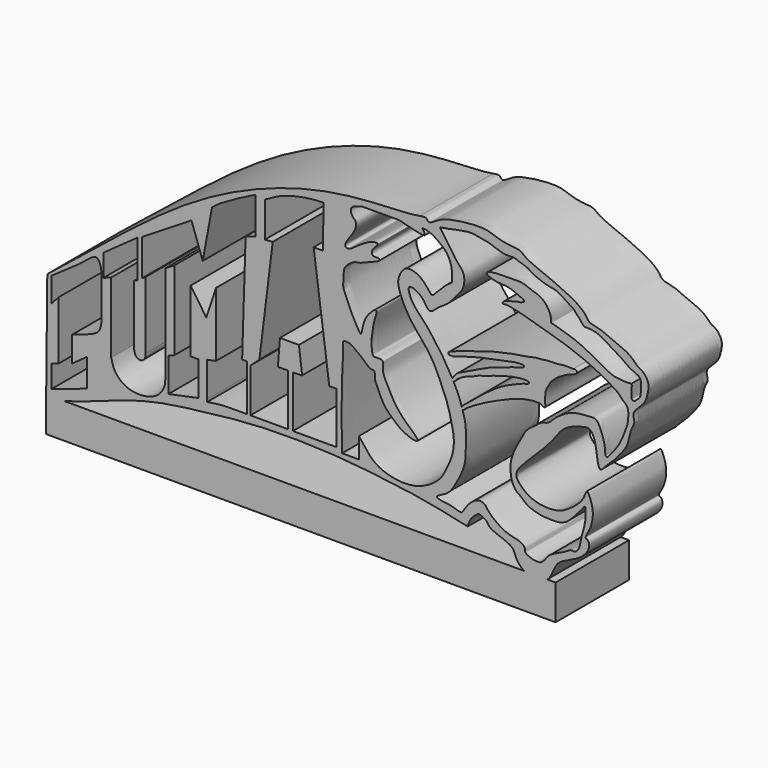
from build123d import *

# Parameters (mm, degrees)
F1_DEPTH = 20
F2_W     = 111.0479156588
F2_H     = 7.6344155701
F3_DEPTH = 20


with BuildPart() as f1:
    # F0 (on Front) → F1 (new body)
    with BuildSketch(Plane.XZ):
        with BuildLine():
            add(Edge.make_bspline(
                [(-68.5763731599, -24.029718712), (-62.8424740639, -19.4761018218), (-51.2870427359, -9.9741760052), (-32.577207567, 3.8970302083), (-8.5290191206, 12.8961252081), (9.7086163121, 13.0013621624), (12.0042391692, 13.4216141178), (12.6355951652, 13.5370446369)],
                knots=[0, 0, 0, 0, 0.2305075204, 0.4671476986, 0.7203497781, 0.9230047089, 1, 1, 1, 1], degree=3))
            Line((-68.5763731599, -24.029718712), (-68.8400990123, -49.0021140309))
            Line((-68.8400990123, -49.0021140309), (-67.2818273306, -47.8710122406))
            add(Edge.make_bspline(
                [(-67.2818273306, -47.8710122406), (-61.0936873368, -46.3664774949), (-49.1456948203, -41.1773982467), (-35.9901500826, -39.5859325488), (-23.4933828008, -38.0194479617), (-7.9544184747, -38.0854578186), (4.0351011583, -39.3360079001), (13.9875895572, -40.6665019925), (20.1001078469, -42.0224792595), (23.0631544298, -42.6801430644)],
                knots=[0, 0, 0, 0, 0.1748702622, 0.3187366349, 0.459197766, 0.6158479055, 0.754475325, 0.8794420979, 1, 1, 1, 1], degree=3))
            ThreePointArc((23.0631544298, -42.6801430644), (23.9464490144, -40.7759790038), (25.5563499174, -39.429030907))
            add(Edge.make_bspline(
                [(25.5563499174, -39.429030907), (26.1716625414, -39.6596022431), (27.3518612756, -40.1044976448), (27.7137964068, -41.7947097929), (33.1747303772, -42.9476295263), (33.3915021172, -45.4281539159), (35.7692568103, -48.0598457762), (41.3055342618, -47.9927628403), (41.9812373993, -42.883346931), (46.4047970825, -41.7440891079), (49.7857335986, -38.9620867614), (49.4956044988, -36.6956066003), (48.363130973, -36.5804430799), (49.9309341811, -34.6064106874), (50.5213747284, -31.4169708175), (50.108031679, -29.3425503211), (49.0232752449, -26.6090951701), (48.4739110603, -29.5594445155), (45.1258995017, -32.2008787119), (42.6546621411, -33.4876654823), (38.9384909011, -33.4863281815), (36.339694077, -32.5510247197), (34.2587013719, -30.8460209421), (33.14465329, -28.8158671071), (36.3034997793, -25.5921561608), (39.625862845, -22.3717114064), (41.6447003496, -20.0915280792), (43.0394886465, -17.9829548722), (44.9649642471, -16.270024253), (48.1341514666, -15.3318192091), (49.8205409339, -15.0591641924), (51.2193543877, -17.5815222843), (51.4579236491, -23.513175539), (53.1785046157, -21.1480303175), (54.7164859754, -19.9741312742), (56.5790834553, -17.6703813705), (58.1932679013, -15.5653781875), (58.4560193303, -12.5331844032), (59.7591870259, -10.8853380525), (58.5829563084, -9.0027633437), (61.709761443, -6.8157320682), (62.2784459421, -4.5471949838), (62.7867288075, -2.1367958021), (61.0445580767, -0.2100928655), (60.2541340875, -0.0851524026), (59.4746538103, 0.7961116283), (57.9762840665, 2.1258575397), (54.7069320423, 3.3546083874), (52.2854621802, 4.6056235075), (49.4149561727, 4.9542350847), (48.9835662994, 6.2526229564), (46.680608127, 8.2529520546), (43.1362195894, 9.7788813803), (41.6027546429, 10.5205784164), (39.6470245398, 11.3299557773), (37.4213779274, 12.1396946885), (35.4958827322, 13.1736840083), (34.3536675322, 14.2578538304), (31.7790832126, 14.2057000076), (28.8726627219, 15.0299179873), (27.1131732469, 15.7523169184), (23.3109314875, 15.6544083262), (19.399034179, 15.0975749866), (16.7432067765, 14.2594341947), (14.9146380272, 12.8093572388), (14.2668846406, 13.1623013209), (14.0411098054, 13.7738687719), (13.1720313766, 13.627432199), (12.6355951652, 13.5370446369)],
                knots=[0, 0, 0, 0, 0.0128906595, 0.0246453603, 0.0460755988, 0.0603354354, 0.0777175692, 0.0981562797, 0.1177821882, 0.1378619387, 0.1576052625, 0.170275515, 0.1777469708, 0.19122827, 0.2088810173, 0.2238704146, 0.236935849, 0.2498612246, 0.2700920494, 0.286410647, 0.3045313212, 0.3206836367, 0.3363322107, 0.3493730315, 0.3688889221, 0.3903022143, 0.407043062, 0.4220983379, 0.4376305213, 0.4551207774, 0.4665194786, 0.4826922908, 0.5034058812, 0.5151812999, 0.5294625771, 0.5458845909, 0.5616833513, 0.5782965055, 0.5915054006, 0.6038100797, 0.6213156282, 0.6362732181, 0.6510407179, 0.665696027, 0.6740429806, 0.6839305184, 0.6976067432, 0.7155841904, 0.7321442087, 0.7476178336, 0.7579985815, 0.7747019213, 0.7938175182, 0.8064582323, 0.8202405581, 0.8353452595, 0.8495036912, 0.8611660563, 0.8763967251, 0.893141174, 0.9064170318, 0.92499084, 0.944463415, 0.9608928393, 0.9748715551, 0.981946496, 0.9888043556, 1, 1, 1, 1], degree=3))
        make_face()
        with BuildLine():
            Line((-67.6202252507, -29.3487161398), (-67.6202252507, -24.029718712))
            add(Edge.make_bspline(
                [(-63.15773819, -33.9078567922), (-61.5074046053, -33.3753877232), (-58.8261670773, -32.5103088081), (-57.1355470776, -31.3741286232), (-56.6463044332, -29.3712492055), (-56.7989735672, -25.0925295019), (-56.5854431257, -19.2767948952), (-57.3062910621, -17.7206121949), (-58.1642828184, -17.0182992197), (-60.3673849688, -18.9638502975), (-64.6799909941, -22.1019544197), (-67.6202252507, -24.029718712)],
                knots=[0, 0, 0, 0, 0.1344522729, 0.21810492, 0.301110973, 0.4329190842, 0.5837822348, 0.6615185097, 0.714935113, 0.8099422179, 1, 1, 1, 1], degree=3))
            Line((-63.15773819, -33.9078567922), (-63.15773819, -39.4494543357))
            Line((-63.15773819, -39.4494543357), (-59.9204339087, -37.0995940954))
            Line((-59.9204339087, -37.0995940954), (-59.9204339087, -43.2110093534))
            Line((-59.9204339087, -43.2110093534), (-67.681632936, -45.812278986))
            Line((-67.681632936, -45.812278986), (-67.681632936, -40.9478149984))
            Line((-67.681632936, -40.9478149984), (-66.1323964596, -40.4285676777))
            Line((-66.1323964596, -40.4285676777), (-66.1323964596, -27.7001184301))
            Line((-66.1323964596, -27.7001184301), (-67.6202252507, -29.3487161398))
        make_face(mode=Mode.SUBTRACT)
        with BuildLine():
            Line((-56.3480295241, -20.7848474383), (-56.3480295241, -15.9424301237))
            Line((-56.3480295241, -15.9424301237), (-48.9367544651, -10.6603609944))
            Line((-48.9367544651, -10.6603609944), (-48.9367544651, -18.8947413117))
            Line((-48.9367544651, -18.8947413117), (-49.6612451971, -19.1793628672))
            Line((-49.6612451971, -19.1793628672), (-49.6612451971, -32.3095694184))
            add(Edge.make_bspline(
                [(-49.6612451971, -32.3095694184), (-49.550913704, -32.5792308171), (-49.4735777947, -33.3253336595), (-48.9232087266, -33.8958631419), (-47.8595334721, -34.0964704749), (-47.1028458665, -33.0518824561), (-47.1613099679, -32.5387496049), (-47.1861027181, -32.3095694184)],
                knots=[0, 0, 0, 0, 0.2109435836, 0.3940078694, 0.5974043108, 0.8207649572, 1, 1, 1, 1], degree=3))
            Line((-47.1861027181, -32.3095694184), (-47.1861027181, -17.6569670439))
            Line((-47.1861027181, -17.6569670439), (-47.9423962533, -18.1223899126))
            Line((-47.9423962533, -18.1223899126), (-47.9423962533, -10.2101974189))
            Line((-47.9423962533, -10.2101974189), (-37.1425785124, -3.4970382694))
            Line((-37.1425785124, -3.4970382694), (-34.6929617226, -10.4895886034))
            Line((-34.6929617226, -10.4895886034), (-32.6580479741, 0.4966819542))
            add(Edge.make_bspline(
                [(-32.6580479741, 0.4966819542), (-31.6459829579, 1.3301714982), (-29.8156036109, 2.5123849062), (-26.2045528268, 4.4330040138), (-24.1211841262, 5.55334523), (-23.2389662415, 5.9331734665)],
                knots=[0, 0, 0, 0, 0.3299609283, 0.6827711276, 1, 1, 1, 1], degree=3))
            Line((-23.2389662415, 5.9331734665), (-23.2389662415, -2.0397095941))
            Line((-23.2389662415, -2.0397095941), (-25.3467336297, -2.7791610919))
            Line((-25.3467336297, -2.7791610919), (-26.1013221078, -26.6294348985))
            Line((-26.1013221078, -26.6294348985), (-25.0671431422, -26.6294348985))
            Line((-25.0671431422, -26.6294348985), (-25.0671431422, -36.741334945))
            add(Edge.make_bspline(
                [(-25.0671431422, -36.741334945), (-26.3252303884, -36.7258496034), (-28.7008392181, -36.6966090922), (-31.6308565733, -36.8875220527), (-33.0835662989, -37.1412270736), (-33.7508358061, -37.2577607632)],
                knots=[0, 0, 0, 0, 0.378372384, 0.7144693495, 1, 1, 1, 1], degree=3))
            Line((-33.7508358061, -37.2577607632), (-33.7640754879, -36.741334945))
            Line((-33.7640754879, -36.741334945), (-33.7640754879, -29.138345798))
            Line((-33.7640754879, -29.138345798), (-31.794089824, -28.7411157042))
            Line((-31.794089824, -28.7411157042), (-31.794089824, -14.7206289694))
            Line((-31.794089824, -14.7206289694), (-33.918403089, -21.0935790092))
            Line((-33.918403089, -21.0935790092), (-37.3236909509, -16.0667231292))
            Line((-37.3236909509, -16.0667231292), (-37.3236909509, -29.6698175371))
            Line((-37.3236909509, -29.6698175371), (-35.660982132, -29.6698175371))
            Line((-35.660982132, -29.6698175371), (-35.660982132, -37.109284196))
            Line((-35.660982132, -37.109284196), (-42.1798937023, -38.4673907732))
            Line((-42.1798937023, -38.4673907732), (-42.1798937023, -31.0817323625))
            Line((-42.1798937023, -31.0817323625), (-40.8984795213, -30.6096319109))
            Line((-40.8984795213, -30.6096319109), (-40.8984795213, -13.3854517873))
            Line((-40.8984795213, -13.3854517873), (-42.8405329585, -14.5506840199))
            Line((-42.8405329585, -14.5506840199), (-42.8405329585, -35.5389267206))
            add(Edge.make_bspline(
                [(-54.6512380242, -35.5389267206), (-54.4245839545, -36.4442620263), (-53.931170017, -38.415129165), (-50.5420565368, -40.9685900651), (-45.2064643534, -40.5118258501), (-42.9223532416, -37.8091151365), (-42.8659685902, -36.2446646398), (-42.8405329585, -35.5389267206)],
                knots=[0, 0, 0, 0, 0.1836112314, 0.3997119522, 0.644773585, 0.8397541172, 1, 1, 1, 1], degree=3))
            Line((-54.6512380242, -35.5389267206), (-54.6512380242, -20.1670583338))
            Line((-54.6512380242, -20.1670583338), (-56.3480295241, -20.7848474383))
        make_face(mode=Mode.SUBTRACT)
        with BuildLine():
            Line((-21.1528521031, -2.0069417078), (-21.1528521031, 5.7083428837))
            add(Edge.make_bspline(
                [(-21.1528521031, 5.7083428837), (-20.1003651535, 6.3187885742), (-17.9155580527, 7.5859834595), (-13.7988873339, 8.7460943954), (-10.4805822381, 9.2007744218), (-9.0379980514, 9.2152428669), (-8.4088556468, 9.2215528712)],
                knots=[0, 0, 0, 0, 0.2663248992, 0.5528510649, 0.8049886039, 1, 1, 1, 1], degree=3))
            Line((-8.4088556468, 9.2215528712), (-8.4274644032, 0))
            Line((-8.4274644032, 0), (-10.5071477592, 0))
            Line((-10.5071477592, 0), (-7.1003274061, -25.5388338119))
            Line((-7.1003274061, -25.5388338119), (-5.4923477583, -25.5388338119))
            Line((-5.4923477583, -25.5388338119), (-5.4923477583, -36.741334945))
            Line((-5.4923477583, -36.741334945), (-15.0402951986, -36.741334945))
            Line((-15.0402951986, -36.741334945), (-15.0402951986, -25.47673136))
            Line((-15.0402951986, -25.47673136), (-13.0293034017, -25.410797447))
            Line((-13.0293034017, -25.410797447), (-13.7177789584, -19.7872146964))
            Line((-13.7177789584, -19.7872146964), (-17.861418426, -19.7872146964))
            Line((-17.861418426, -19.7872146964), (-18.3040369302, -25.47673136))
            Line((-18.3040369302, -25.47673136), (-16.0689745098, -25.47673136))
            Line((-16.0689745098, -25.47673136), (-16.0689745098, -36.741334945))
            Line((-16.0689745098, -36.741334945), (-24.2825746536, -36.741334945))
            Line((-24.2825746536, -36.741334945), (-24.2825746536, -27.1698180586))
            Line((-24.2825746536, -27.1698180586), (-22.335955239, -25.410797447))
            Line((-22.335955239, -25.410797447), (-19.4306913763, -1.869168831))
            Line((-19.4306913763, -1.869168831), (-21.1528521031, -2.0069417078))
        make_face(mode=Mode.SUBTRACT)
        with BuildLine():
            add(Edge.make_bspline(
                [(13.1149329245, 11.4469267428), (13.2454424113, 11.265540442), (13.5017344209, 10.9093375275), (14.0798250427, 9.9265843409), (11.9921920887, 10.3150667891), (9.3961707003, 10.8682942314), (8.3365435753, 11.3562675048), (5.2628460876, 11.1676267303), (1.4134467959, 11.2473589646), (0.0227734326, 11.3111626559), (-0.8636605807, 10.8570442048), (-1.9383073615, 10.6542583041), (-2.4270764263, 10.1920794525), (-2.4098521462, 9.325496849), (-1.936654468, 8.4605651843), (-1.2957633129, 8.1106285788), (-1.1941500149, 6.5018633305), (-2.3064935859, 5.0299367339), (-3.2934459387, 3.6039608268), (-3.7530027477, 2.6985577325), (-3.363455326, 2.0513797894), (-2.2784933492, 2.3048448469), (-0.6581018721, 3.7386091033), (1.1914715646, 4.671528638), (2.0996055947, 5.2467896361), (4.0963186692, 5.4843413959), (2.4310462008, 3.9496448812), (2.057302188, 3.2403916948), (2.4101538771, 2.334543307), (3.6449311374, 2.5977628138), (3.9979083618, 2.2141175488), (3.3495048099, 1.6984931235), (1.7460088106, 1.2415812933), (-0.3552107945, 0.1699458693), (-1.698762065, 0.1970740724), (-3.4454235187, -1.1434876811), (-4.0011264115, -2.1229225594), (-4.0193230978, -4.5170312493), (-4.1669284386, -5.7428791166), (-2.8987263025, -8.3243099324), (-2.1297921371, -10.3240843808), (-0.6548038421, -12.8414710721), (-0.2276660592, -13.4580342627), (0.0556774798, -12.6325087625), (0.2337403686, -11.4435931249), (0.6618419334, -10.2191982524), (1.269346609, -9.1390326043), (2.1484826433, -8.231889505), (2.5779945286, -7.8418971873), (2.8517618261, -7.6601574257), (3.1762750434, -7.5546178135), (3.2616173012, -8.2027558151), (2.7811510965, -9.4209664527), (2.4302861584, -10.9923666744), (2.2550789719, -12.4495099501), (2.0075769976, -13.7766201014), (2.1885419282, -15.7747065486), (2.4751401995, -16.889099067), (3.4669993278, -16.6221565323), (4.2346679021, -16.7619717693), (4.7779826125, -17.0446088063), (4.3344533036, -19.0130874806), (5.721595114, -21.4741059315), (6.9664758787, -24.0776386974), (9.2151011375, -26.8092605363), (10.6988688311, -27.9292142464), (11.7172701448, -28.9657842684), (12.4404026364, -29.8329394905), (11.3742229698, -30.0095697484), (9.9356421891, -29.4498423173), (8.4618387431, -28.8139448721), (6.6323109237, -27.1865886424), (5.0062867854, -25.6943605934), (3.8998537977, -23.5413761077), (3.2636028786, -21.9867176539), (2.7069994861, -20.915651109), (2.9770063005, -19.252616312), (1.7969919761, -19.4229915113), (0.9098473053, -18.5047254773), (-0.6092325432, -17.2494448742), (-1.533446625, -16.6011797284), (-2.487423885, -15.8622744104), (-3.2908907548, -15.860254335), (-4.2504746017, -15.6163677239), (-4.019144832, -18.0375390004), (-4.3630860957, -22.2375592594), (-4.5214006905, -31.2084520815), (-4.3110004626, -37.5204570591)],
                knots=[0, 0, 0, 0, 0.0083871544, 0.0164688024, 0.0288112058, 0.0453967227, 0.0558365001, 0.0729670657, 0.0926563772, 0.1039508445, 0.1135550149, 0.1237527145, 0.13132907, 0.1401639553, 0.1497659263, 0.1577698247, 0.1693629384, 0.1828971777, 0.1960573939, 0.2055387359, 0.2127473388, 0.2221709698, 0.2369159506, 0.2510110489, 0.2619725466, 0.2725744132, 0.2847141685, 0.2940190896, 0.3022983772, 0.3127711078, 0.318330634, 0.3260539625, 0.3391321531, 0.3541499816, 0.3656172875, 0.3796016841, 0.3902381501, 0.4050102041, 0.4162654288, 0.4323176585, 0.4477357949, 0.4645012583, 0.4710358037, 0.4787105679, 0.4899162886, 0.5011140579, 0.5121907721, 0.5232303057, 0.5306436192, 0.5362746619, 0.5410445653, 0.5478224262, 0.5592434936, 0.5719266364, 0.5837295601, 0.5952873087, 0.6094166969, 0.6188578498, 0.627894564, 0.6366829551, 0.6432552251, 0.6562065851, 0.6727181209, 0.689834476, 0.7082012397, 0.72167869, 0.7337849309, 0.7424898352, 0.7507036997, 0.763097174, 0.7756890099, 0.7909391309, 0.8057673206, 0.8210006386, 0.833695512, 0.8446836397, 0.8559755358, 0.8648145789, 0.8758904082, 0.8897518873, 0.9004813451, 0.910936758, 0.9198801755, 0.927739317, 0.9408486915, 0.9609068341, 1, 1, 1, 1], degree=3))
            add(Edge.make_bspline(
                [(-0.6561594782, -33.0408181175), (-0.035652913, -33.8626542442), (1.2155842949, -35.5198674437), (3.5168527453, -37.8087591992), (7.9171780503, -39.0052123015), (11.7615988371, -38.7653015247), (14.5901260849, -37.533092362), (17.2156468794, -35.5901900018), (18.4976848628, -33.040918417), (19.8691271694, -30.1235870757), (20.2123975557, -26.7733900062), (19.5213175063, -23.6446639212), (18.6349047357, -20.2435125181), (17.6216857054, -17.9922458122), (15.6772356677, -13.3418208854), (13.2887033228, -10.2949847948), (10.7071343576, -7.3843904229), (8.8028686978, -4.1077386098), (7.7185245302, -1.0489519232), (8.1235728753, 0.8410546592), (9.4328177043, 2.799162206), (11.7395616106, 2.5336595786), (13.6792742589, 1.2327935868), (15.1922757938, -1.0484076658), (15.6880826756, -0.5522752558), (16.7707954606, 0.5779130569), (17.5241453321, 1.3605404433), (18.4301937149, 2.2307846442), (19.7242244397, 2.9620222635), (19.6149120897, 3.5342651834), (19.6917472385, 5.0038971788), (19.5024920618, 6.4153707199), (18.562032301, 8.497381305), (17.3070456925, 9.5000557411), (16.2776299305, 10.2762086716), (15.2740757169, 10.9309394715), (14.1412753371, 11.2924457196), (13.4495642164, 11.3966113586), (13.1149329245, 11.4469267428)],
                knots=[0, 0, 0, 0, 0.0322707381, 0.0650399499, 0.1038618123, 0.1398422198, 0.1719327954, 0.2045717184, 0.2354578959, 0.2683741304, 0.3017219568, 0.3349580476, 0.3688298157, 0.3981956437, 0.4389760175, 0.4757398142, 0.5117346155, 0.5479236801, 0.5803814755, 0.6055638571, 0.6320217353, 0.6579864657, 0.68734805, 0.7155466683, 0.7275571363, 0.7506067352, 0.7702509745, 0.7912750478, 0.8126057944, 0.8254268821, 0.8472173537, 0.8698461488, 0.8972195022, 0.9205493959, 0.9412780642, 0.9613483157, 0.9812982559, 1, 1, 1, 1], degree=3))
            Line((-0.6561594782, -33.0408181175), (-0.6561594782, -37.5204570591))
            Line((-0.6561594782, -37.5204570591), (-4.3110004626, -37.5204570591))
        make_face(mode=Mode.SUBTRACT)
        with BuildLine():
            add(Edge.make_bspline(
                [(17.0841336351, 12.7163172), (17.816161154, 11.6189452677), (19.1604477338, 9.6037474088), (20.6664432108, 7.3766720753), (22.3273993151, 5.8987675251), (22.3922207189, 3.6564091781), (21.8762247664, 2.0662007346), (19.8418630574, 0.0014335713), (18.8093748214, -1.4393306047), (16.5299443556, -2.6010367842), (14.7165509382, -4.7535042616), (13.5811906867, -2.2747865343), (12.2092411584, -1.2496068888), (11.0771416619, -0.6529574777), (9.8924641815, -0.7954449334), (10.6646527097, -3.1397247399), (11.9635149006, -4.8476877258), (14.0809259567, -6.8496355128), (16.4279645117, -10.0984268825), (17.6050110376, -11.769082258), (18.7496305182, -13.5767852663), (19.5360881146, -14.9832356329), (19.7466184679, -15.3735313595)],
                knots=[0, 0, 0, 0, 0.0093192229, 0.0171427526, 0.0240747115, 0.0308814227, 0.0370874622, 0.0450740315, 0.0514910318, 0.0592530711, 0.0661419814, 0.072887806, 0.079364404, 0.084724767, 0.0888693687, 0.0956151997, 0.1028282485, 0.1110450608, 0.1205682043, 0.1274133905, 0.135536896, 0.1385735761, 0.1385735761, 0.1385735761, 0.1385735761], degree=3))
            add(Edge.make_bspline(
                [(58.7086154351, -3.7098187022), (58.7575826978, -3.7638790664), (58.8801513344, -3.8991881436), (58.7910363742, -4.4402645372), (58.7984741188, -5.3751263327), (58.827958268, -6.2617494256), (58.7948619909, -6.6305001059), (59.023329139, -6.804572873), (59.419611634, -6.8195402864), (59.7205652029, -6.5973420149), (60.2618346637, -6.0927991422), (60.7810410992, -5.5238539958), (60.8377062719, -3.9874344052), (60.9149850635, -2.7600201737), (60.6335143592, -1.8824163864), (60.0588257828, -1.5117752223), (58.9051608413, -1.0406365304), (57.9045532683, -0.4783762414), (56.960296564, 0.2823810251), (56.372079104, 0.6558442358), (55.2364788399, 1.2875888185), (54.3585193901, 1.8877445624), (53.2848558449, 2.5497152391), (52.3615543424, 3.1321344463), (51.4897467898, 3.5136861858), (50.9092580092, 3.749535455), (50.1176164563, 3.8410651041), (49.1976692589, 3.9647302334), (48.6161478337, 3.8671370765), (48.3046605591, 4.1092904634), (47.8773003267, 4.4956294027), (47.4484080765, 5.2442345638), (46.740666053, 5.7640741683), (46.4357579422, 6.357542198), (45.8073218371, 6.810852867), (44.7552248108, 7.4451028528), (44.3673871829, 7.7093556556), (42.4701726692, 9.0448684169), (40.6611159434, 9.1058567867), (38.7132354371, 9.8441851555), (37.1997335101, 10.3881195268), (35.9960736002, 11.4177012251), (33.9643685252, 11.8495216408), (33.4325128393, 12.2505204309), (31.9566459365, 12.1783752773), (31.0754964675, 12.1965069011), (30.3087553781, 12.3822129666), (29.0440085637, 12.7601261379), (27.8975701844, 13.2911933304), (26.3540810585, 13.5165327709), (25.2937772269, 13.7127334798), (23.9007007887, 14.006713945), (22.0831354351, 13.7632054074), (20.3348467077, 13.4574687334), (19.0715778274, 13.0810325578), (17.7861806483, 12.9760156267), (17.2958679619, 12.7946453974), (17.0841336351, 12.7163172)],
                knots=[0, 0, 0, 0, 0.0086815097, 0.0217294282, 0.0400641548, 0.0575678905, 0.0681013381, 0.0771420047, 0.0882535158, 0.0993912764, 0.1150075426, 0.1309374985, 0.1534185133, 0.1743643813, 0.191119142, 0.2058959575, 0.2262785846, 0.2465590233, 0.266404454, 0.282005101, 0.302626303, 0.3220275248, 0.3425651169, 0.3620512832, 0.3797988096, 0.3942186767, 0.4106213396, 0.4285912517, 0.4422475538, 0.4531627477, 0.4669907378, 0.4841679055, 0.5013090904, 0.5158889746, 0.5323107728, 0.5522437279, 0.5655477651, 0.5924996252, 0.617961924, 0.6442183688, 0.6673603309, 0.6907647298, 0.7165811017, 0.7317131116, 0.7534632882, 0.7710177596, 0.7871074328, 0.8080429008, 0.8291476789, 0.8518529928, 0.8710599312, 0.8926616362, 0.9177481055, 0.942325045, 0.9636508351, 0.9843029605, 1, 1, 1, 1], degree=3))
            add(Edge.make_bspline(
                [(21.9570909853, -20.7023481974), (22.1617589553, -21.3451488475), (22.6255232655, -22.8545369616), (22.7628290276, -25.6850734761), (22.6044800653, -28.0524002222), (22.6630482648, -30.4810375624), (21.5756577584, -33.4289443176), (20.0774748785, -35.9052863937), (18.9399977193, -37.8942372624), (15.4264245939, -39.1611910228), (17.9375925547, -39.721482251), (19.5198153114, -39.7373460793), (21.7712222623, -40.7086491695), (22.1466773594, -39.8277220362), (23.1113128662, -38.4368667816), (24.0604874875, -37.5582384963), (25.2245033713, -36.7678866859), (26.773701419, -36.9661776917), (27.337202975, -38.0319782715), (28.5355602565, -39.2300801802), (29.7903036803, -40.1087975205), (31.3594197944, -41.0971273889), (32.9858494114, -41.4896303823), (34.785620179, -41.8553639259), (35.669664357, -42.7585421075), (35.4200260861, -43.6525324507), (36.6345797405, -44.133082294), (37.4080152648, -44.4595841819), (38.2734166908, -44.4398327569), (38.8863049383, -44.5017944242), (39.5539669693, -43.913984267), (39.9609931934, -43.6254855134), (40.4076708062, -42.6206470559), (42.0098513468, -41.6657050799), (43.3994366477, -41.0906560239), (44.785396748, -40.3213785416), (45.6164080501, -39.7677540186), (46.521235683, -40.0753950665), (47.2010057415, -39.2846746891), (47.5863294053, -38.4496625974), (47.7603901725, -36.7879551259), (48.3298418898, -35.2087307299), (48.5829920289, -33.9366407383), (48.8248997891, -32.6139479335), (48.7103626047, -31.3591021858), (48.8564791682, -30.6326217849), (48.5254651263, -30.4647876306), (48.1395884555, -31.1395609068), (47.5051630068, -31.7427461907), (46.6685071707, -32.838201186), (45.8140316113, -33.6537172631), (44.742550321, -34.7849723935), (43.7873997524, -35.1260370174), (43.1741337502, -35.4179251215), (41.8160349428, -35.4988036781), (40.5457155629, -35.4245411176), (39.134472636, -35.380796386), (37.881417918, -35.0319141641), (35.9338162559, -34.5023477853), (34.5922306293, -32.9525786188), (33.63937814, -32.5986030857), (32.7592339443, -31.115529487), (32.4586710582, -29.7401843279), (32.2696559612, -27.6786463417), (32.9518422537, -25.3892704061), (33.8239690305, -23.5770851636), (34.5318488814, -22.4781228728), (35.7189885129, -19.7652427926), (37.8928997811, -18.590705731), (39.0444794975, -17.3759520562), (40.7222385304, -17.2328282235), (41.8935065092, -15.7457985042), (43.6702551243, -14.4788553747), (45.3601794339, -13.520263261), (47.6249410087, -13.0104254186), (49.5398729125, -12.9804483669), (51.2136074746, -12.7141080475), (52.1251924565, -14.7361568064), (52.7086575632, -16.3746917208), (53.0762249851, -18.0843830926), (53.0422896471, -18.9931056505), (53.1158657774, -19.4635210054), (53.6816728465, -19.4550884439), (54.0061010095, -18.8387070718), (55.0555889082, -17.6514805797), (55.9463576285, -16.5062941165), (56.8954553882, -14.5585533584), (57.3412382773, -13.2828068298), (57.9441292253, -11.8173539235), (58.0609639819, -10.5692680316), (58.1402321195, -9.5256235493), (57.9583809654, -8.4775964297), (57.4685176773, -7.8970873717), (56.4808773462, -7.1451034441), (55.9651990755, -6.3409974695), (54.7425324129, -5.6311905423), (53.700542636, -4.9262028922), (52.0373160004, -3.9942087316), (50.5566739963, -3.3819793865), (48.4313147557, -2.2753733998), (46.7621464075, -1.8186019666), (44.7600525663, -0.9349911706), (43.0184715759, -0.3616440676), (40.0660248213, 0.4117238381), (38.9206011294, 0.8349585322), (37.19369387, 1.2552655679), (35.5683277256, 1.7441253504), (34.3198411783, 2.1256253149), (32.5317827325, 2.4056760321), (31.7233291036, 2.7301000951), (30.4397630983, 2.425161342), (30.9454199565, 3.2371337753), (31.813785914, 3.4477145651), (32.5207381284, 3.6538955757), (33.2678070342, 3.8194494394), (34.030521615, 4.064703185), (34.6223321118, 4.0591448265), (35.0683845205, 4.2955191024), (35.3944926818, 4.4514003975), (35.3626372612, 4.820600675), (34.6648119617, 5.0653313881), (33.8600526418, 5.4723733718), (33.0484340527, 5.8037602198), (31.9182266524, 6.1223758841), (30.7645751371, 6.285963445), (29.7105502774, 6.2660929675), (28.8708156015, 6.4612986785), (28.0946639595, 6.6666021541), (27.5831612412, 6.9748291234), (26.9632451016, 7.1638703367), (27.4622135024, 7.5956330707), (28.0324474284, 7.8062835435), (29.0695933516, 7.8943681245), (29.5886365979, 8.0016184079), (31.3452914813, 7.9513601066), (33.0337283392, 7.9969053119), (35.0875005651, 8.0779291486), (37.0152531251, 7.2188692107), (38.6184437488, 6.7633449226), (39.9123503189, 5.8758508046), (40.5178514487, 5.0144087489), (40.9631915911, 4.2483765607), (41.2853137372, 3.2676299862), (41.1874292427, 2.2056239193), (41.5571983026, 2.2824667118), (42.4420747207, 2.0632094857), (43.8452983351, 1.5362562125), (45.8290187598, 1.0533515843), (48.2710237653, -0.0028069515), (50.2076646979, -0.979686875), (52.8579240991, -2.5610829894), (54.0924406999, -3.1036408094), (54.8597335523, -3.4664090693), (55.8024361178, -3.5617820029), (57.151861267, -3.7312988694), (58.214317647, -3.7463954724), (58.5033871177, -3.6448721746), (58.7086154351, -3.7098187022)],
                knots=[0.154076916, 0.154076916, 0.154076916, 0.154076916, 0.1604338558, 0.1686540911, 0.1760206587, 0.1833923163, 0.1918310154, 0.1999162943, 0.2074824736, 0.2150247112, 0.2206649716, 0.2274229643, 0.234302321, 0.2383369787, 0.2445443436, 0.2500880898, 0.2556445742, 0.261209507, 0.2663056063, 0.2724669321, 0.2784634613, 0.2848835029, 0.2911359087, 0.297607561, 0.3026162291, 0.3066646435, 0.3117320196, 0.3162811746, 0.3206142582, 0.3243187901, 0.328654389, 0.33202434, 0.3368288578, 0.3433004019, 0.34931393, 0.3553066376, 0.3599485706, 0.3642412809, 0.3687732633, 0.3733850397, 0.3795253509, 0.3857689771, 0.3911971538, 0.3967344654, 0.4021946716, 0.4060556379, 0.4081915445, 0.4120732983, 0.416717891, 0.4222513795, 0.4275675692, 0.4334952301, 0.4382070565, 0.4420990935, 0.4475691685, 0.4530885058, 0.4586707774, 0.4641322013, 0.4709004716, 0.4775982613, 0.482347539, 0.4883704056, 0.4941150428, 0.5008981018, 0.5083587711, 0.5150135102, 0.5205243496, 0.5285781357, 0.5360809093, 0.5421092739, 0.5479901514, 0.5544321626, 0.5614858278, 0.5681700714, 0.5753962166, 0.5821086629, 0.5878251907, 0.5944573835, 0.6010140618, 0.6072908575, 0.6118389292, 0.6147523282, 0.617787635, 0.6216484371, 0.6276074436, 0.6335466478, 0.6404834154, 0.6461516793, 0.6520889144, 0.6574354224, 0.6623482983, 0.6671353861, 0.6712769029, 0.6765116765, 0.6812211626, 0.6867566628, 0.6922305106, 0.6987176965, 0.7049055408, 0.7122005493, 0.7186013361, 0.7254919897, 0.7322031742, 0.7404273176, 0.745828421, 0.7520989824, 0.7583318977, 0.7638935656, 0.7701983925, 0.7749477345, 0.7794794102, 0.7829619919, 0.7875834281, 0.7917034012, 0.7958848359, 0.8001592846, 0.8038110521, 0.807192057, 0.8099026808, 0.8123107695, 0.8162679364, 0.8208855762, 0.8253632475, 0.8305251725, 0.8357274452, 0.8406114974, 0.8450516369, 0.8492826981, 0.8531326883, 0.8563287603, 0.859478011, 0.8634222551, 0.8681694903, 0.8717396257, 0.8779020596, 0.8843021215, 0.8910785469, 0.8979824622, 0.9041981149, 0.9100887774, 0.9149375397, 0.9193725288, 0.9243934041, 0.9288955796, 0.9311693971, 0.9356253175, 0.9415158745, 0.9484054213, 0.9561234005, 0.9633684177, 0.9717288638, 0.9772697175, 0.9814988928, 0.9861136182, 0.9917949446, 0.9966167011, 1, 1, 1, 1], degree=3))
            add(Edge.make_bspline(
                [(21.9570909853, -20.7023481974), (21.8208919987, -20.6704850624), (21.7481580687, -20.4076465648), (21.7940676265, -20.1904542275)],
                knots=[0.8582463589, 0.8582463589, 0.8582463589, 0.8582463589, 0.8761910068, 0.8761910068, 0.8761910068, 0.8761910068], degree=3))
            add(Edge.make_bspline(
                [(19.9922965947, -15.8356707543), (20.3642188153, -16.5459456468), (21.1689233892, -18.2007091586), (21.566658039, -19.4725497982), (21.7940676265, -20.1904542275)],
                knots=[0.1397651489, 0.1397651489, 0.1397651489, 0.1397651489, 0.1452370777, 0.1523821316, 0.1523821316, 0.1523821316, 0.1523821316], degree=3))
            add(Edge.make_bspline(
                [(19.9922965947, -15.8356707543), (19.852087546, -15.8074308364), (19.7357965237, -15.5513096348), (19.7466184679, -15.3735313595)],
                knots=[0.3656944081, 0.3656944081, 0.3656944081, 0.3656944081, 0.3736191076, 0.3736191076, 0.3736191076, 0.3736191076], degree=3))
        make_face(mode=Mode.SUBTRACT)
        with BuildLine():
            add(Edge.make_bspline(
                [(19.7466184679, -15.3735313595), (19.7563954016, -15.2129200687), (19.9925271261, -15.0118526837), (20.2357270855, -14.5647686216), (20.8381076243, -13.9119725205), (21.9515051005, -13.4243501064), (22.8304236117, -12.9378645774), (24.1019289097, -12.4237719299), (24.8599502327, -12.0921791688), (25.6545365971, -11.5904723485), (26.641734467, -11.1998666449), (27.755317055, -10.6235760145), (28.8799283042, -10.2744476988), (29.8303176504, -9.9933900871), (30.7406923758, -9.6443264378), (31.7146055534, -9.349746023), (32.653943817, -8.9642121722), (33.5177069765, -8.7158882615), (34.3724607086, -8.4968829807), (34.8987238254, -8.3083960898), (35.2270360463, -8.2004245532), (35.4041741347, -7.9930538375), (35.2784693813, -7.7207488299), (34.8297665524, -7.7073967305), (33.8865551054, -7.7512951076), (32.9862104462, -7.8337572266), (31.4288724821, -8.2334856854), (29.7275900586, -8.4798847099), (28.0031569065, -8.9904198412), (25.3033251102, -9.3903442678), (23.2691774545, -10.0900609699), (21.5833418453, -10.4879010419), (19.9682170106, -11.1383770258), (19.4063650872, -11.0271682649), (18.8916003127, -11.0860231529), (18.7656177482, -10.5463989698), (19.4971153463, -10.2836468266), (20.4382757609, -9.8786891549), (21.7070757376, -9.4576670895), (23.1832230647, -8.9718562902), (24.4066627691, -8.6333438044), (26.2621732627, -8.0492073655), (27.5309510441, -7.6394783808), (28.8992472873, -7.2016249025), (30.3049384264, -6.9545823718), (31.9368614098, -6.6072204821), (33.121873409, -6.278445343), (34.7733609487, -5.9928277413), (36.428639314, -5.8337207254), (37.7030780487, -5.3871812737), (39.2211020612, -5.4131549829), (40.0353947133, -5.1811697665), (41.5320977278, -5.1594821043), (42.725199755, -5.1247892639), (44.0265484252, -4.8643566503), (45.2282947053, -4.9207543744), (45.8155365346, -4.9311467085), (46.0829214662, -4.9358785447)],
                knots=[0.3736191076, 0.3736191076, 0.3736191076, 0.3736191076, 0.3807785662, 0.3885106197, 0.3987181729, 0.4107168921, 0.4219509911, 0.4346470615, 0.4446975928, 0.4551150437, 0.4664428938, 0.478752251, 0.4906549332, 0.5015298856, 0.5123018081, 0.5233790766, 0.5343977545, 0.5448673797, 0.5551688363, 0.5633499611, 0.5696959563, 0.5749518486, 0.5801071431, 0.5870954103, 0.5977023103, 0.6082635048, 0.6220398016, 0.6364117015, 0.6511588112, 0.6692596151, 0.6853744999, 0.7000556408, 0.714173845, 0.7224000673, 0.7295638587, 0.7360743351, 0.745002666, 0.7562963146, 0.7690600656, 0.782606618, 0.7951519488, 0.8102986408, 0.8231355235, 0.8360483836, 0.849289684, 0.8633207767, 0.8755418966, 0.8896670128, 0.9038055075, 0.9166484079, 0.9298211143, 0.9400354647, 0.9531988767, 0.9653882937, 0.9779559206, 0.9899656051, 1, 1, 1, 1], degree=3))
            add(Edge.make_bspline(
                [(19.7466184679, -15.3735313595), (19.829229156, -15.5266807655), (19.9113064362, -15.6810005761), (19.9922965947, -15.8356707543)],
                knots=[0.1385735761, 0.1385735761, 0.1385735761, 0.1385735761, 0.1397651489, 0.1397651489, 0.1397651489, 0.1397651489], degree=3))
            add(Edge.make_bspline(
                [(25.651739918, -16.8306766873), (25.8456873814, -16.6868938165), (26.2407282348, -16.3940213402), (26.8189775625, -15.8579038568), (27.549652966, -15.3719148745), (28.3308215553, -14.8231015935), (29.1327352311, -14.2135554759), (29.956333793, -13.7170974221), (30.5768412608, -13.3409856327), (31.3711301016, -12.9155152945), (32.3030842047, -12.5000579204), (33.2332621558, -12.0672366895), (34.0041558505, -11.819395615), (34.6461273112, -11.5439643236), (35.2188274869, -11.2832990792), (35.7137063806, -11.1897354315), (36.1540612699, -11.0364559878), (36.4399887436, -10.9131023289), (36.4369293889, -10.634860706), (36.1786135074, -10.4788304821), (35.7404405471, -10.4799002677), (34.9344687838, -10.4052881666), (33.9282611265, -10.6198068084), (32.6499795904, -10.7445873954), (32.0305088278, -11.0187110058), (31.1026873591, -11.1086428474), (30.2171594702, -11.5035742973), (29.2453690962, -11.7141635574), (28.4969337078, -11.9817743773), (27.4483821799, -12.369155176), (26.6019878654, -12.5688982496), (25.837524714, -12.8160051236), (25.0635987111, -13.0937456285), (24.2068740977, -13.5199471501), (23.6520324782, -13.6901506317), (22.7826433864, -13.964582237), (21.9353448234, -14.3780074208), (21.3675482641, -14.7696667078), (20.6041300206, -15.2158749378), (20.1656443454, -15.8705852359), (19.9922965947, -15.8356707543)],
                knots=[0, 0, 0, 0, 0.0093501937, 0.0190497617, 0.0292969486, 0.04001892, 0.0510944429, 0.0617806344, 0.0710916797, 0.0814003675, 0.0925728891, 0.1036944495, 0.1135431609, 0.1226879854, 0.131325198, 0.1391240442, 0.1466500582, 0.1524263441, 0.157485267, 0.1630742668, 0.170245882, 0.1799777673, 0.1913438463, 0.2036490379, 0.2126714163, 0.2230101357, 0.23391654, 0.2447192815, 0.2545732394, 0.2660933217, 0.2763963198, 0.2860853462, 0.2961464942, 0.3067406916, 0.3151313598, 0.325534721, 0.3361925507, 0.3452275443, 0.3558966893, 0.3656944081, 0.3656944081, 0.3656944081, 0.3656944081], degree=3))
            add(Edge.make_bspline(
                [(21.7940676265, -20.1904542275), (21.852880695, -19.9122170055), (22.3775918149, -19.4913950835), (23.1553149404, -18.8839812406), (23.9669913059, -18.2153448978), (24.9153713241, -17.45139123), (25.4162249716, -17.0291979499), (25.651739918, -16.8306766873)],
                knots=[0.8761910068, 0.8761910068, 0.8761910068, 0.8761910068, 0.8991792441, 0.9237694994, 0.9489998899, 0.9760213378, 1, 1, 1, 1], degree=3))
            add(Edge.make_bspline(
                [(21.7940676265, -20.1904542275), (21.8116895365, -20.2460844556), (21.865670277, -20.4163260458), (21.9203516242, -20.5869608938), (21.9570909853, -20.7023481974)],
                knots=[0.1523821316, 0.1523821316, 0.1523821316, 0.1523821316, 0.1529357999, 0.154076916, 0.154076916, 0.154076916, 0.154076916], degree=3))
            add(Edge.make_bspline(
                [(46.0829214662, -4.9358785447), (46.2396704671, -4.9042102549), (46.5628004158, -4.8389291902), (47.1047323081, -5.3355276984), (46.5592950224, -5.8451121643), (45.6426692939, -6.1252917396), (44.4406048154, -6.5777897613), (43.354327297, -7.2935004947), (42.6229613667, -7.6529667996), (41.9010132242, -8.3631178037), (41.1422407101, -8.9962695169), (40.7228394673, -9.9422314265), (40.1083384345, -10.8080393026), (39.9880325746, -11.7711792348), (39.948450164, -12.4964785916), (39.9137630632, -13.2330067201), (40.0906850593, -14.5298591709), (39.4668384683, -14.2609952782), (39.1644912134, -14.0477933769), (38.7557815532, -13.8695915168), (37.8687133099, -13.9453974187), (37.5864631367, -13.8546642695), (36.8262508291, -13.990739359), (36.1185205218, -14.1188432018), (35.2918965329, -14.2418669053), (34.3954048506, -14.4463425819), (33.2490690682, -14.951257337), (32.6605181504, -15.0306496868), (31.7728529394, -15.4765942176), (30.8750660779, -15.7625328015), (30.0275071932, -16.2014215414), (29.0952904806, -16.6045206809), (28.0407126405, -17.1269877444), (27.0813076858, -17.5407969265), (26.1948123814, -18.0866154595), (25.371624862, -18.4533789372), (24.6349123751, -18.9231998689), (23.7263313258, -19.5204171259), (22.7752266385, -19.9412822671), (22.1432658927, -20.7459029725), (21.9570909853, -20.7023481974)],
                knots=[0, 0, 0, 0, 0.0169248575, 0.0348909269, 0.0531640707, 0.0774684819, 0.1055620033, 0.1333599511, 0.1554166031, 0.1797326627, 0.2040218091, 0.2287316731, 0.2539269162, 0.2777436506, 0.2981909493, 0.3205650316, 0.3453132581, 0.3609532393, 0.3763364194, 0.392670425, 0.4152805261, 0.4289830788, 0.4497680118, 0.4710883309, 0.4930922666, 0.5170779036, 0.5441036626, 0.5631567822, 0.5870453861, 0.6111177922, 0.6348372944, 0.6595889448, 0.6861401692, 0.7113153376, 0.7362001795, 0.7593234402, 0.7821591659, 0.807381869, 0.8337172252, 0.8582463589, 0.8582463589, 0.8582463589, 0.8582463589], degree=3))
        make_face()
        with BuildLine():
            add(Edge.make_bspline(
                [(19.7466184679, -15.3735313595), (19.829229156, -15.5266807655), (19.9113064362, -15.6810005761), (19.9922965947, -15.8356707543)],
                knots=[0.1385735761, 0.1385735761, 0.1385735761, 0.1385735761, 0.1397651489, 0.1397651489, 0.1397651489, 0.1397651489], degree=3))
            add(Edge.make_bspline(
                [(19.9922965947, -15.8356707543), (19.852087546, -15.8074308364), (19.7357965237, -15.5513096348), (19.7466184679, -15.3735313595)],
                knots=[0.3656944081, 0.3656944081, 0.3656944081, 0.3656944081, 0.3736191076, 0.3736191076, 0.3736191076, 0.3736191076], degree=3))
        make_face()
        with BuildLine():
            add(Edge.make_bspline(
                [(21.9570909853, -20.7023481974), (21.8208919987, -20.6704850624), (21.7481580687, -20.4076465648), (21.7940676265, -20.1904542275)],
                knots=[0.8582463589, 0.8582463589, 0.8582463589, 0.8582463589, 0.8761910068, 0.8761910068, 0.8761910068, 0.8761910068], degree=3))
            add(Edge.make_bspline(
                [(21.7940676265, -20.1904542275), (21.8116895365, -20.2460844556), (21.865670277, -20.4163260458), (21.9203516242, -20.5869608938), (21.9570909853, -20.7023481974)],
                knots=[0.1523821316, 0.1523821316, 0.1523821316, 0.1523821316, 0.1529357999, 0.154076916, 0.154076916, 0.154076916, 0.154076916], degree=3))
        make_face()
    extrude(amount=F1_DEPTH)

    # F2 (on face) → F3 (join)
    with BuildSketch(Plane.XZ.offset(20)):
        with Locations((-13.2970621395, -51.0127131359)):
            Rectangle(F2_W, F2_H)
    extrude(amount=-F3_DEPTH)


solid = f1.part
